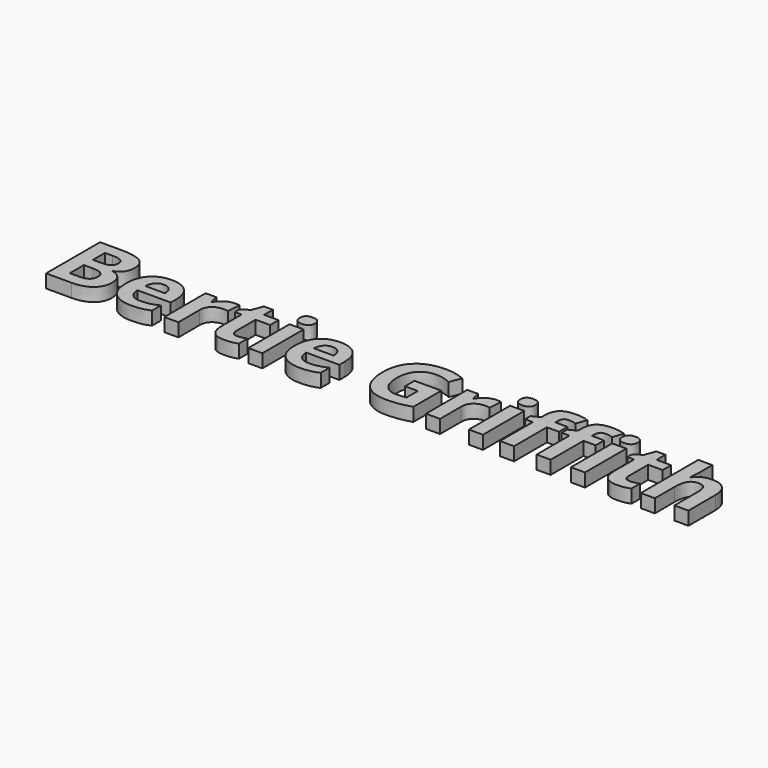
from build123d import *

# Parameters (mm, degrees)
F0_TEXT_SIZE = 179.6795262231
F1_DEPTH     = 25.4


# Not quite as in the source:
# - Text() gives the source's letters only with a copy of the font that has no kerning and outlines rounded to 1/6400 em; it was checked with that copy


with BuildPart() as f1:
    # F0 (on Top) → F1 (new body)
    with BuildSketch(Plane.XY):
        with Locations((-207.0181071758, 64.2852634192)):
            Text('Bertie Griffith', F0_TEXT_SIZE, font='Open Sans', font_style=FontStyle.BOLD, text_align=(TextAlign.LEFT, TextAlign.BOTTOM))
    extrude(amount=F1_DEPTH)


solid = f1.part
